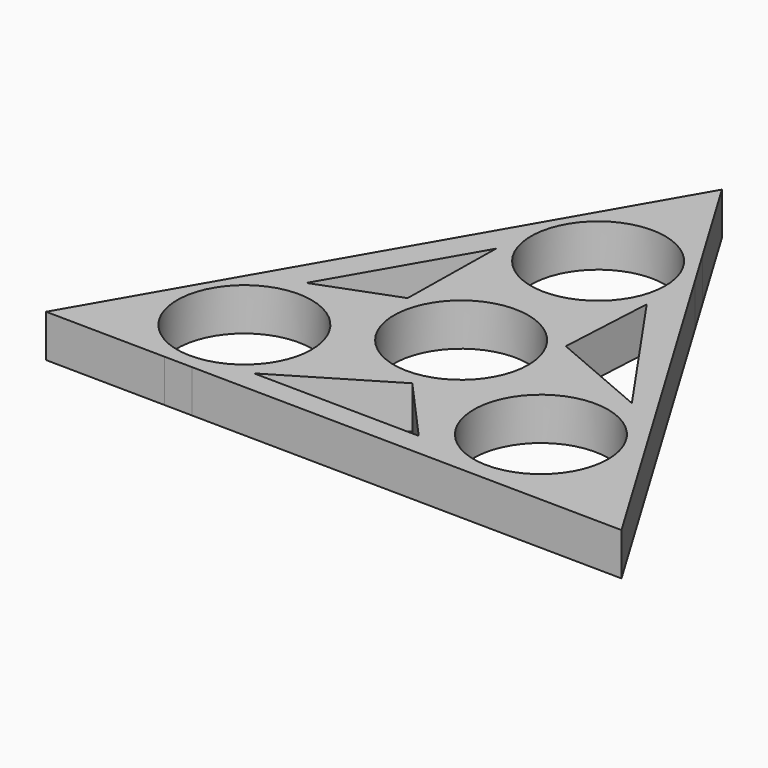
from build123d import *

# Parameters (mm, degrees)
F0_R     = 11.05
F0_R_2   = 13.55
F1_DEPTH = 7


with BuildPart() as f1:
    # F0 (on Top) → F1 (new body)
    with BuildSketch(Plane.XY):
        with BuildLine():
            ThreePointArc((2.6065338711, -13.2969350295), (10.4623380263, -8.6105739079), (13.55, 0))
            ThreePointArc((13.55, 0), (13.0425271945, 3.6735520114), (11.5581203867, 7.0719412559))
            ThreePointArc((11.5581203867, 7.0719412559), (-1.2547280417, 13.4917811108), (-12.6639989198, 4.8192978077))
            ThreePointArc((-12.6639989198, 4.8192978077), (-10.3603872444, -8.7329763624), (2.6065338711, -13.2969350295))
        make_face()
        Circle(F0_R, mode=Mode.SUBTRACT)
        with BuildLine():
            ThreePointArc((11.5581203867, 7.0719412559), (13.0425271945, 3.6735520114), (13.55, 0))
            ThreePointArc((13.55, 0), (10.4623380263, -8.6105739079), (2.6065338711, -13.2969350295))
            Line((2.6065338711, -13.2969350295), (12.3875978298, -24.2038302976))
            Line((12.3875978298, -24.2038302976), (-14.9941514566, -23.8444135863))
            ThreePointArc((-14.9941514566, -23.8444135863), (-18.3532690256, -26.2108119603), (-22.267239092, -27.461551912))
            Line((-22.267239092, -27.461551912), (49.0895092572, -28.3981906763))
            Line((49.0895092572, -28.3981906763), (13.0464962981, 31.8175852156))
            ThreePointArc((13.0464962981, 31.8175852156), (13.4235339021, 30.0051079331), (13.55, 28.1581543386))
            ThreePointArc((13.55, 28.1581543386), (13.2562145915, 25.351862354), (12.3875978298, 22.6672600574))
            Line((12.3875978298, 22.6672600574), (28.0773907901, 0))
            Line((28.0773907901, 0), (11.5581203867, 7.0719412559))
        make_face()
        with Locations((24.3843801233, -14.0799748264)):
            Circle(F0_R_2, mode=Mode.SUBTRACT)
        with BuildLine():
            ThreePointArc((-12.6639989198, 4.8192978077), (-1.2547280417, 13.4917811108), (11.5581203867, 7.0719412559))
            Line((11.5581203867, 7.0719412559), (12.3875978298, 22.6672600574))
            ThreePointArc((12.3875978298, 22.6672600574), (0, 14.6081543386), (-12.3875978298, 22.6672600574))
            Line((-12.3875978298, 22.6672600574), (-12.6639989198, 4.8192978077))
        make_face()
        with BuildLine():
            Line((-14.9941514566, -23.8444135863), (2.6065338711, -13.2969350295))
            ThreePointArc((2.6065338711, -13.2969350295), (-10.3603872444, -8.7329763624), (-12.6639989198, 4.8192978077))
            Line((-12.6639989198, 4.8192978077), (-25.4531481717, 0))
            Line((-25.4531481717, 0), (-12.3875978298, 22.6672600574))
            ThreePointArc((-12.3875978298, 22.6672600574), (-13.4461101823, 26.4834540771), (-13.3560221409, 30.4427051857))
            Line((-13.3560221409, 30.4427051857), (-32.9787461707, -3.600513583))
            ThreePointArc((-32.9787461707, -3.600513583), (-18.5911674875, -1.8305608799), (-10.8371028035, -14.0784028862))
            ThreePointArc((-10.8371028035, -14.0784028862), (-11.9196052449, -19.3853798623), (-14.9941514566, -23.8444135863))
        make_face()
        with BuildLine():
            ThreePointArc((-12.3875978298, 22.6672600574), (0, 14.6081543386), (12.3875978298, 22.6672600574))
            ThreePointArc((12.3875978298, 22.6672600574), (13.2562145915, 25.351862354), (13.55, 28.1581543386))
            ThreePointArc((13.55, 28.1581543386), (13.4235339021, 30.0051079331), (13.0464962981, 31.8175852156))
            Line((13.0464962981, 31.8175852156), (9.3890984881, 37.9278692567))
            ThreePointArc((9.3890984881, 37.9278692567), (0.4816570964, 41.6995909847), (-8.6712487219, 38.5702600624))
            Line((-8.6712487219, 38.5702600624), (-13.3560221409, 30.4427051857))
            ThreePointArc((-13.3560221409, 30.4427051857), (-13.4461101823, 26.4834540771), (-12.3875978298, 22.6672600574))
        make_face()
        with Locations((0, 28.1581543386)):
            Circle(F0_R, mode=Mode.SUBTRACT)
        with BuildLine():
            ThreePointArc((-22.267239092, -27.461551912), (-18.3532690256, -26.2108119603), (-14.9941514566, -23.8444135863))
            ThreePointArc((-14.9941514566, -23.8444135863), (-11.9196052449, -19.3853798623), (-10.8371028035, -14.0784028862))
            ThreePointArc((-10.8371028035, -14.0784028862), (-18.5911674875, -1.8305608799), (-32.9787461707, -3.600513583))
            Line((-32.9787461707, -3.600513583), (-37.7601482446, -11.895708306))
            ThreePointArc((-37.7601482446, -11.895708306), (-35.4713085242, -21.872174986), (-26.8575138424, -27.4012993168))
            Line((-26.8575138424, -27.4012993168), (-22.267239092, -27.461551912))
        make_face()
        with Locations((-24.3871028035, -14.0784028862)):
            Circle(F0_R, mode=Mode.SUBTRACT)
        with BuildLine():
            Line((-46.5486845968, -27.1428302263), (-26.8575138424, -27.4012993168))
            ThreePointArc((-26.8575138424, -27.4012993168), (-35.4713085242, -21.872174986), (-37.7601482446, -11.895708306))
            Line((-37.7601482446, -11.895708306), (-46.5486845968, -27.1428302263))
        make_face()
        with BuildLine():
            Line((0, 53.6139011383), (-8.6712487219, 38.5702600624))
            ThreePointArc((-8.6712487219, 38.5702600624), (0.4816570964, 41.6995909847), (9.3890984881, 37.9278692567))
            Line((9.3890984881, 37.9278692567), (0, 53.6139011383))
        make_face()
        with Locations((24.3843801233, -14.0799748264)):
            Circle(F0_R_2)
        with Locations((24.3843801233, -14.0799748264)):
            Circle(F0_R, mode=Mode.SUBTRACT)
    extrude(amount=F1_DEPTH)


solid = f1.part
